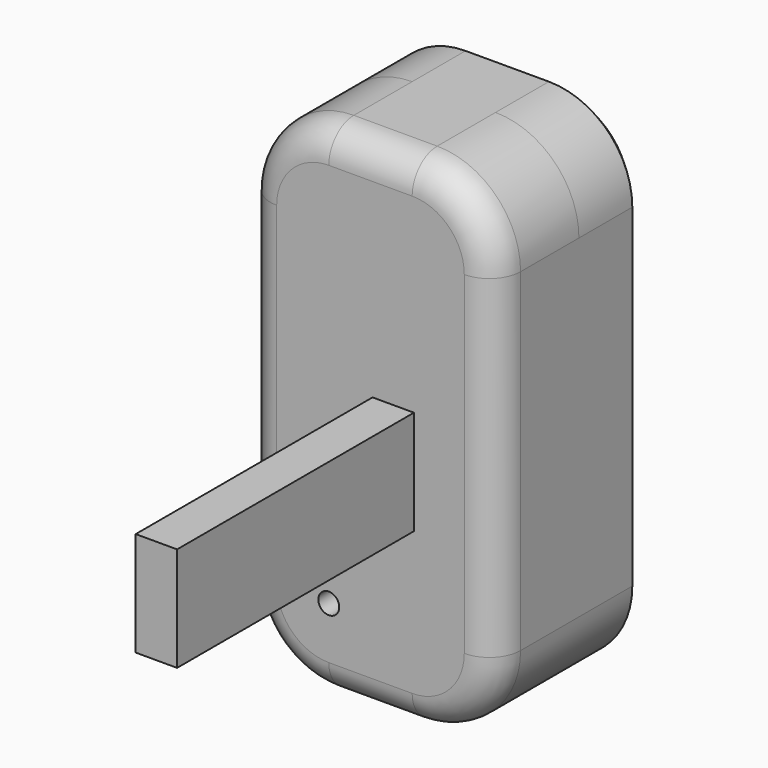
from build123d import *

# Parameters (mm, degrees)
F0_W      = 152.4
F0_H      = 50.8
F1_DEPTH  = 304.8
F2_R      = 50.8
F3_DEPTH  = 63.5
F4_T      = -12.7
F9_SIZE   = 10.16
F10_R     = 6.35
F5_DEPTH  = 114.301
F7_R      = 19.05
F6_W      = 25.2215266228
F6_H      = 63.5711848736
F11_DEPTH = 180.3614813834


# Not quite as in the source:
# - a feature names something its author has since deleted; it is built from what else it names


with BuildPart() as f1:
    # F0 (on Top) → F1 (new body)
    with BuildSketch(Plane.XY):
        with Locations((76.2, 25.4)):
            Rectangle(F0_W, F0_H)
    extrude(amount=F1_DEPTH)

    # F2
    f2_edges = [f1.edges().sort_by_distance(p)[0] for p in [
        (152.4, 25.4, 304.8),
        (152.4, 25.4, 0),
        (0, 25.4, 304.8),
        (0, 25.4, 0),
    ]]
    fillet(f2_edges, radius=F2_R)

    # F3 (add): a face of the model
    f3_faces = [f1.faces().sort_by_distance(p)[0] for p in [
        (76.2, 0, 152.4),
    ]]
    extrude(f3_faces, amount=F3_DEPTH)

    # F4
    f4_openings = [f1.faces().sort_by_distance(p)[0] for p in [
        (76.2, 50.8, 152.4),
    ]]
    offset(amount=F4_T, openings=f4_openings)

    # F9
    f9_edges = [f1.edges().sort_by_distance(p)[0] for p in [
        (0, 50.8, 152.4),
        (14.878976, 50.8, 14.878976),
        (137.521024, 50.8, 14.878976),
        (152.4, 50.8, 152.4),
        (137.521024, 50.8, 289.921024),
        (76.2, 50.8, 304.8),
        (76.2, 50.8, 0),
        (14.878976, 50.8, 289.921024),
    ]]
    chamfer(f9_edges, length=F9_SIZE)

    # F10 (on face) → F5 (cut, through all)
    with BuildSketch(Plane(origin=(0, 50.8, 0), x_dir=(-1, 0, 0), z_dir=(0, 1, 0))):
        with Locations((-50.8, 50.8)):
            Circle(F10_R)
    extrude(amount=-F5_DEPTH, mode=Mode.SUBTRACT)

    # F7
    f7_edges = [f1.edges().sort_by_distance(p)[0] for p in [
        (152.4, -63.5, 152.4),
        (0, -63.5, 152.4),
        (14.878976, -63.5, 289.921024),
        (14.878976, -63.5, 14.878976),
        (76.2, -63.5, 0),
        (76.2, -63.5, 304.8),
        (137.521024, -63.5, 14.878976),
        (137.521024, -63.5, 289.921024),
    ]]
    fillet(f7_edges, radius=F7_R)

    # F6 (on face) → F11 (join)
    with BuildSketch(Plane.XZ.offset(63.5)):
        with Locations((90.0648534298, 138.1654888391)):
            Rectangle(F6_W, F6_H)
    extrude(amount=F11_DEPTH)


solid = f1.part
